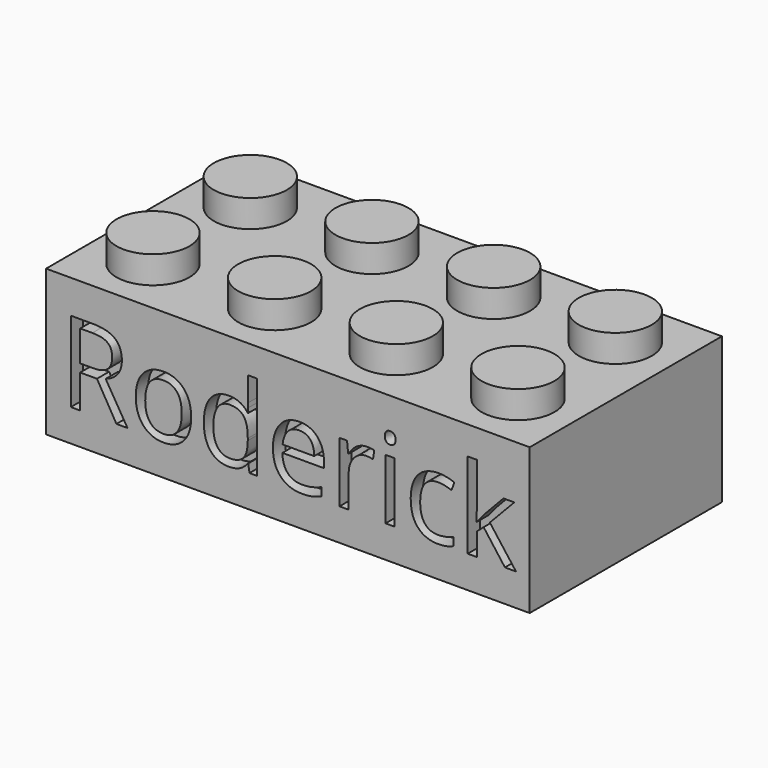
from build123d import *

# Parameters (mm, degrees)
F0_W          = 31.8
F0_H          = 15.8
F1_DEPTH      = 9.6
F2_W          = 29.4
F2_H          = 13.4
F3_DEPTH      = 8.4
F4_R          = 2.4
F5_DEPTH      = 1.8
F6_R          = 1.3
F7_DEPTH      = 1.2
F8_R          = 3.255
F8_R_2        = 2.4
F9_DEPTH      = 8.4
F10_W         = 0.6
F10_H         = 0.3
F11_DEPTH     = 8.4
F12_W         = 0.3
F12_H         = 0.6
F13_DEPTH     = 8.4
F14_W         = 0.6
F14_H         = 4
F15_DEPTH     = 6.4
F16_TEXT_SIZE = 7.4116965837
F17_DEPTH     = 1


# Not quite as in the source:
# - a feature names something its author has since deleted; it is built from what else it names
# - Text() gives the source's letters only with a copy of the font that has no kerning and outlines rounded to 1/6400 em; it was checked with that copy


with BuildPart() as f1:
    # F0 (on Top) → F1 (new body)
    with BuildSketch(Plane.XY):
        Rectangle(F0_W, F0_H)
    extrude(amount=F1_DEPTH)

    # F2 (on face) → F3 (cut)
    with BuildSketch(Plane(origin=(0, 0, 0), x_dir=(1, 0, 0), z_dir=(0, 0, -1))):
        Rectangle(F2_W, F2_H)
    extrude(amount=-F3_DEPTH, mode=Mode.SUBTRACT)

    # F4 (on face) → F5 (join)
    with BuildSketch(Plane.XY.offset(9.6)):
        with Locations((-11.95, 3.95)):
            Circle(F4_R)
        with Locations((-3.95, 3.95)):
            Circle(F4_R)
        with Locations((4.05, 3.95)):
            Circle(F4_R)
        with Locations((12.05, 3.95)):
            Circle(F4_R)
        with Locations((12.05, -4.05)):
            Circle(F4_R)
        with Locations((4.05, -4.05)):
            Circle(F4_R)
        with Locations((-3.95, -4.05)):
            Circle(F4_R)
        with Locations((-11.95, -4.05)):
            Circle(F4_R)
    extrude(amount=F5_DEPTH)

    # F6 (on face) → F7 (cut)
    with BuildSketch(Plane(origin=(0, 0, 8.4), x_dir=(1, 0, 0), z_dir=(0, 0, -1))):
        with Locations((-11.95, 3.95)):
            Circle(F6_R)
        with Locations((-11.95, -4.05)):
            Circle(F6_R)
        with Locations((-3.95, 3.95)):
            Circle(F6_R)
        with Locations((-3.95, -4.05)):
            Circle(F6_R)
        with Locations((4.05, 3.95)):
            Circle(F6_R)
        with Locations((4.05, -4.05)):
            Circle(F6_R)
        with Locations((12.05, 3.95)):
            Circle(F6_R)
        with Locations((12.05, -4.05)):
            Circle(F6_R)
    extrude(amount=-F7_DEPTH, mode=Mode.SUBTRACT)

    # F8 (on face) → F9 (join, through all)
    with BuildSketch(Plane(origin=(0, 0, 8.4), x_dir=(1, 0, 0), z_dir=(0, 0, -1))):
        with Locations((-7.95, -0.05)):
            Circle(F8_R)
        with Locations((-7.95, -0.05)):
            Circle(F8_R_2, mode=Mode.SUBTRACT)
        with Locations((0.05, -0.05)):
            Circle(F8_R)
        with Locations((0.05, -0.05)):
            Circle(F8_R_2, mode=Mode.SUBTRACT)
        with Locations((8.05, -0.05)):
            Circle(F8_R)
        with Locations((8.05, -0.05)):
            Circle(F8_R_2, mode=Mode.SUBTRACT)
    extrude(amount=F9_DEPTH)

    # F10 (on face) → F11 (join, through all)
    with BuildSketch(Plane(origin=(0, 0, 0), x_dir=(1, 0, 0), z_dir=(0, 0, -1))):
        with Locations((-11.95, 6.55)):
            Rectangle(F10_W, F10_H)
        with Locations((-11.95, -6.55)):
            Rectangle(F10_W, F10_H)
        with Locations((-3.95, 6.55)):
            Rectangle(F10_W, F10_H)
        with Locations((-3.95, -6.55)):
            Rectangle(F10_W, F10_H)
        with Locations((4.05, 6.55)):
            Rectangle(F10_W, F10_H)
        with Locations((4.05, -6.55)):
            Rectangle(F10_W, F10_H)
        with Locations((12.05, 6.55)):
            Rectangle(F10_W, F10_H)
        with Locations((12.05, -6.55)):
            Rectangle(F10_W, F10_H)
    extrude(amount=-F11_DEPTH)

    # F12 (on face) → F13 (join, through all)
    with BuildSketch(Plane(origin=(0, 0, 8.4), x_dir=(1, 0, 0), z_dir=(0, 0, -1))):
        with Locations((-14.55, 3.95)):
            Rectangle(F12_W, F12_H)
        with Locations((-14.55, -4.05)):
            Rectangle(F12_W, F12_H)
        with Locations((14.55, 3.95)):
            Rectangle(F12_W, F12_H)
        with Locations((14.55, -4.05)):
            Rectangle(F12_W, F12_H)
    extrude(amount=F13_DEPTH)

    # F14 (on face) → F15 (join)
    with BuildSketch(Plane(origin=(0, 0, 8.4), x_dir=(1, 0, 0), z_dir=(0, 0, -1))):
        with Locations((0, 4.7)):
            Rectangle(F14_W, F14_H)
        with Locations((0, -4.7)):
            Rectangle(F14_W, F14_H)
    extrude(amount=F15_DEPTH)

    # F16 (on face) → F17 (cut)
    with BuildSketch(Plane.XZ.offset(7.9)):
        with Locations((-15, 2.1135784598)):
            Text('Roderick', F16_TEXT_SIZE, font='Open Sans', text_align=(TextAlign.LEFT, TextAlign.BOTTOM))
    extrude(amount=-F17_DEPTH, mode=Mode.SUBTRACT)


solid = f1.part
